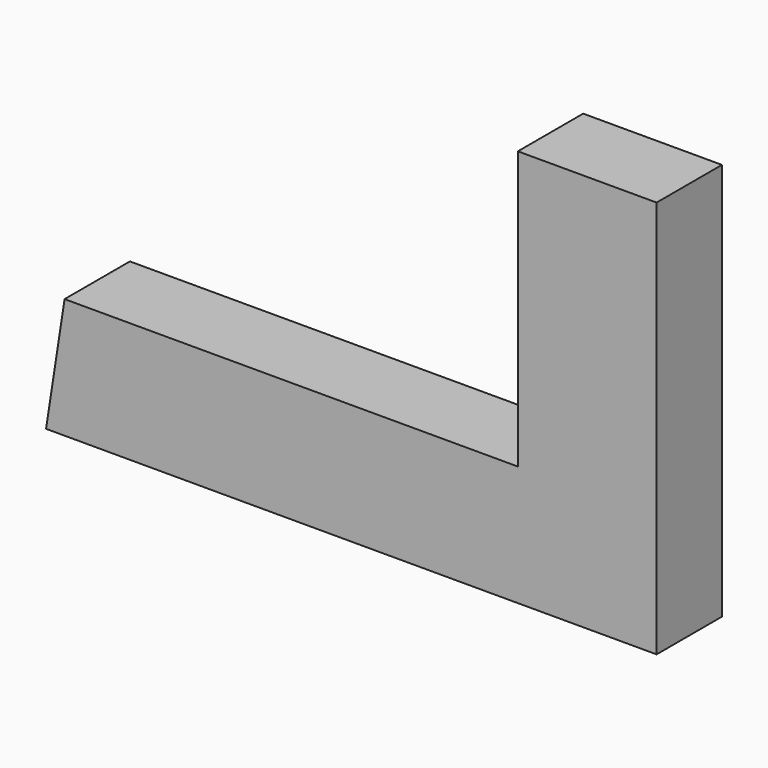
from build123d import *

# Parameters (mm, degrees)
F1_DEPTH = 2.54
F2_R     = 2.6712032827
F3_DEPTH = 2.54


# Not quite as in the source:
# - the program builds the solid bodies; features that only make, move or delete a surface that nothing else refers to are left out


with BuildPart() as f1:
    # F0 (on Front) → F1 (new body)
    with BuildSketch(Plane.XZ):
        Polygon((-38.4220704436, 27.1976441145), (-38.9976799488, 23.4561692923), (-20.0024992228, 23.4561692923), (-20.0024992228, 35.8318164945), (-24.3195872754, 35.8318164945), (-24.3195872754, 31.2269236892), (-24.3195872754, 27.1976441145), align=None)
    extrude(amount=F1_DEPTH)

    # F2 (on Right) → F3 (cut)
    with BuildSketch(Plane.YZ):
        with Locations((0, 48.1319762766)):
            Circle(F2_R)
    extrude(amount=-F3_DEPTH, mode=Mode.SUBTRACT)


solid = f1.part
